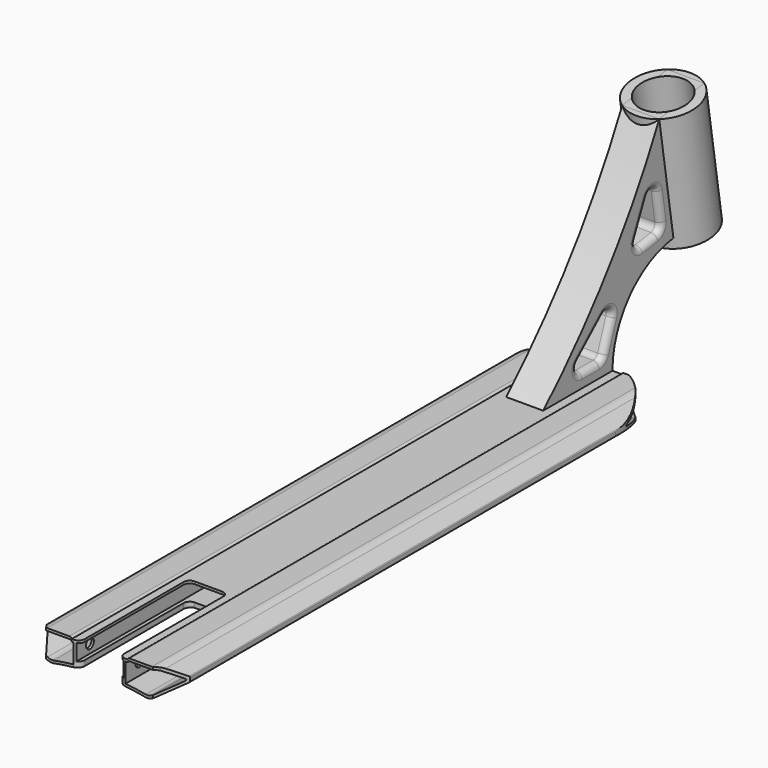
from build123d import *

# Parameters (mm, degrees)
F1_DEPTH       = 250
F2_W           = 38
F2_H           = 13
F3_DEPTH       = 250
F4_R           = 9
F5_R           = 1
F6_T1_DEPTH    = 509.3674969976
F8_DEPTH       = 500.001
F10_DEPTH      = 526
F10_DEPTH_BACK = 24.001
F12_DEPTH      = 527
F12_DEPTH_BACK = 24.0010001
F13_F1_R       = 4.9999
F13_F2_R       = 5
F13_F3_R       = 5
F13_F4_R       = 4.9999
F13_F5_R       = 5
F13_F6_R       = 5
F15_DEPTH      = 15
F16_R          = 27.5
F17_DEPTH      = 100
F19_D          = 40
F21_D          = 8
F21_DEPTH      = 50
F21_TIP        = 2.4034424761
F23_DEPTH      = 72.5010001
F24_R          = 5


# Not quite as in the source:
# - a fillet or chamfer that OpenCascade refuses, or shapes differently, is made with other operations: its cross-section is extruded or revolved along the edge and cut away or added
# - a fillet or chamfer is up to 0.001 mm smaller than in the source, because OpenCascade refuses the exact size
# - an extrude ends at something that could not be found from the text; its depth is read off the source's solid


with BuildPart() as f1:
    # F0 (on Front) → F1 (new body, symmetric)
    with BuildSketch(Plane.XZ):
        with BuildLine():
            Line((22.5, 22.7), (0, 22.7))
            Line((0, 22.7), (-22.5, 22.7))
            Line((-22.5, 22.7), (-22.5, 24))
            Line((-22.5, 24), (-45.5824640741, 24))
            Line((-45.5824640741, 24), (-57.5, 14))
            Line((-57.5, 14), (-57.5, 10))
            Line((-57.5, 10), (-40.1794919243, 0))
            ThreePointArc((-40.1794919243, 0), (0, 4.0775448584), (40.1794919243, 0))
            Line((40.1794919243, 0), (57.5, 10))
            Line((57.5, 10), (57.5, 14))
            Line((57.5, 14), (45.5824640741, 24))
            Line((45.5824640741, 24), (22.5, 24))
            Line((22.5, 24), (22.5, 22.7))
        make_face()
    extrude(amount=F1_DEPTH, both=True)

    # F2 (on Front) → F3 (cut, symmetric)
    with BuildSketch(Plane.XZ):
        with Locations((0, 14.2)):
            Rectangle(F2_W, F2_H)
    extrude(amount=F3_DEPTH, both=True, mode=Mode.SUBTRACT)

    # F4
    f4_edges = [f1.edges().sort_by_distance(p)[0] for p in [
        (40.179492, 0, 0),
        (-40.179492, 0, 0),
        (-45.582464, 0, 24),
        (45.582464, 0, 24),
    ]]
    fillet(f4_edges, radius=F4_R)

    # F5
    f5_edges = [f1.edges().sort_by_distance(p)[0] for p in [
        (57.5, 0, 14),
        (57.5, 0, 10),
        (-57.5, 0, 14),
        (-57.5, 0, 10),
    ]]
    fillet(f5_edges, radius=F5_R)

    # F6: fillet of radius 2 on 2 edges, made by hand

    # F6_s2 → F6_t1 (cut)
    with BuildSketch(Plane.XZ.offset(-254.6837484988)):
        with BuildLine():
            ThreePointArc((-22.5, 22.7), (-23.2333239744, 23.6431676725), (-24.3734993995, 24))
            Line((-24.3734993995, 24), (-22.5, 24))
            Line((-22.5, 24), (-22.5, 22.7))
        make_face()
        with BuildLine():
            ThreePointArc((24.3734993995, 24), (23.2333239744, 23.6431676725), (22.5, 22.7))
            Line((22.5, 22.7), (22.5, 24))
            Line((22.5, 24), (24.3734993995, 24))
        make_face()
    extrude(amount=F6_T1_DEPTH, mode=Mode.SUBTRACT)

    # F7 (on face) → F8 (cut, through all)
    with BuildSketch(Plane.XZ.offset(250)):
        with BuildLine():
            Line((-24.3734993995, 22), (-42.3067319657, 22))
            ThreePointArc((-42.3067319657, 22), (-44.7008729689, 21.5778483455), (-46.8062452335, 20.3623111018))
            Line((-46.8062452335, 20.3623111018), (-55.7563117574, 12.8523135826))
            ThreePointArc((-55.7563117574, 12.8523135826), (-56.1097188459, 11.9991133967), (-55.6135241478, 11.2202437356))
            Line((-55.6135241478, 11.2202437356), (-42.1022690923, 3.4195169923))
            ThreePointArc((-42.1022690923, 3.4195169923), (-39.7790673433, 2.5813219392), (-37.3093701274, 2.6021299876))
            ThreePointArc((-37.3093701274, 2.6021299876), (-29.1789785809, 3.9589777355), (-21, 4.9829952574))
            Line((-21, 4.9829952574), (-21, 20.7))
            Line((-21, 20.7), (-22.5, 20.7))
            ThreePointArc((-22.5, 20.7), (-23.2333239744, 21.6431676725), (-24.3734993995, 22))
        make_face()
        with BuildLine():
            Line((21, 20.7), (21, 4.9829952574))
            ThreePointArc((21, 4.9829952574), (29.1789785809, 3.9589777355), (37.3093701274, 2.6021299876))
            ThreePointArc((37.3093701274, 2.6021299876), (39.7790673433, 2.5813219392), (42.1022690923, 3.4195169923))
            Line((42.1022690923, 3.4195169923), (55.6135241478, 11.2202437356))
            ThreePointArc((55.6135241478, 11.2202437356), (56.1097188459, 11.9991133967), (55.7563117574, 12.8523135826))
            Line((55.7563117574, 12.8523135826), (46.8062452335, 20.3623111018))
            ThreePointArc((46.8062452335, 20.3623111018), (44.7008729689, 21.5778483455), (42.3067319657, 22))
            Line((42.3067319657, 22), (24.3734993995, 22))
            ThreePointArc((24.3734993995, 22), (23.2333239744, 21.6431676725), (22.5, 20.7))
            Line((22.5, 20.7), (21, 20.7))
        make_face()
    extrude(amount=-F8_DEPTH, mode=Mode.SUBTRACT)

    # F9 (on Top) → F10 (cut, two sides)
    with BuildSketch(Plane.XY) as f10_sk:
        with BuildLine():
            ThreePointArc((-57.5, 200), (0, 257.5), (57.5, 200))
            Line((57.5, 200), (57.5, 280))
            Line((57.5, 280), (-57.5, 280))
            Line((-57.5, 280), (-57.5, 200))
        make_face()
    extrude(amount=-F10_DEPTH, mode=Mode.SUBTRACT)
    extrude(f10_sk.sketch, amount=F10_DEPTH_BACK, mode=Mode.SUBTRACT)

    # F11 (on Top) → F12 (cut, two sides)
    with BuildSketch(Plane.XY) as f12_sk:
        Polygon((-43.2975540478, -250), (-68, -216), (-68, -346), (68, -346), (68, -216), (43.2975540478, -250), (16, -250), (16, -140), (-16, -140), (-16, -250), align=None)
    extrude(amount=-F12_DEPTH, mode=Mode.SUBTRACT)
    extrude(f12_sk.sketch, amount=F12_DEPTH_BACK, mode=Mode.SUBTRACT)

    # F13: fillet of radius 5 on 8 edges, made by hand

    # F13_f1 (radius 5 in the source; OpenCascade refuses exactly that, so slightly less here)
    f13_f1_edges = [f1.edges().sort_by_distance(p)[0] for p in [
        (16, -250, 5.5682587842),
    ]]
    fillet(f13_f1_edges, radius=F13_F1_R)

    # F13_f2
    f13_f2_edges = [f1.edges().sort_by_distance(p)[0] for p in [
        (16, -140, 5.5682587842),
    ]]
    fillet(f13_f2_edges, radius=F13_F2_R)

    # F13_f3
    f13_f3_edges = [f1.edges().sort_by_distance(p)[0] for p in [
        (16, -140, 21.7),
    ]]
    fillet(f13_f3_edges, radius=F13_F3_R)

    # F13_f4 (radius 5 in the source; OpenCascade refuses exactly that, so slightly less here)
    f13_f4_edges = [f1.edges().sort_by_distance(p)[0] for p in [
        (-16, -250, 21.7),
    ]]
    fillet(f13_f4_edges, radius=F13_F4_R)

    # F13_f5
    f13_f5_edges = [f1.edges().sort_by_distance(p)[0] for p in [
        (-16, -140, 5.5682587842),
    ]]
    fillet(f13_f5_edges, radius=F13_F5_R)

    # F13_f6
    f13_f6_edges = [f1.edges().sort_by_distance(p)[0] for p in [
        (-16, -140, 21.7),
    ]]
    fillet(f13_f6_edges, radius=F13_F6_R)

    # F14 (on Right) → F15 (join, symmetric)
    with BuildSketch(Plane.YZ):
        with BuildLine():
            ThreePointArc((297.3819995028, 182.7), (245.9666940414, 97.362277853), (180, 22.7))
            Line((180, 22.7), (250, 22.7))
            ThreePointArc((250, 22.7), (267.6550746197, 69.1758946867), (311.7145367693, 92.2079211245))
            Line((311.7145367693, 92.2079211245), (313.0254460068, 83.9311659405))
            Line((313.0254460068, 83.9311659405), (358.4591096742, 91.1271513323))
            Line((358.4591096742, 91.1271513323), (342.8156631702, 189.8959853919))
            Line((342.8156631702, 189.8959853919), (297.3819995028, 182.7))
        make_face()
    extrude(amount=F15_DEPTH, both=True)

    # F16 (on face) → F17 (join, through all)
    with BuildSketch(Plane(origin=(0, -20.9512469128, 132.2809669298), x_dir=(1, 0, 0), z_dir=(0, -0.156434465, 0.9876883406))):
        with Locations((0, 345.3013103746)):
            Circle(F16_R)
    extrude(amount=-F17_DEPTH)

    # F19 (through all)
    with Locations(Plane(origin=(0, -20.9512469128, 132.2809669298), x_dir=(1, 0, 0), z_dir=(0, -0.156434465, 0.9876883406))):
        with Locations((0, 345.3013103746)):
            Hole(F19_D / 2)

    # F21 (one way)
    with BuildSketch(Plane.YZ.offset(21)):
        with Locations((-236, 14.9829952574)):
            Circle(F21_D / 2)
    extrude(amount=-F21_DEPTH, mode=Mode.SUBTRACT)
    with Locations(Plane.YZ.offset(21)):
        with Locations((-236, 14.9829952574)):
            with Locations((0, 0, -(F21_DEPTH + F21_TIP / 2))):  # 118° drill point
                Cone(0, F21_D / 2, F21_TIP, mode=Mode.SUBTRACT)

    # F22 (on face) → F23 (cut, through all)
    with BuildSketch(Plane.YZ.offset(15)):
        Polygon((292.844313904, 147.1129445351), (270.3409635007, 97.4199105839), (299.9716137186, 102.1129445351), align=None)
        Polygon((256.378660542, 79), (206, 34), (240, 34), align=None)
    extrude(amount=-F23_DEPTH, mode=Mode.SUBTRACT)

    # F24
    f24_edges = [f1.edges().sort_by_distance(p)[0] for p in [
        (15, 248.18933, 56.5),
        (0, 256.378661, 79),
        (-15, 248.18933, 56.5),
        (0, 240, 34),
        (15, 296.407964, 124.612945),
        (0, 292.844314, 147.112945),
        (-15, 296.407964, 124.612945),
        (0, 299.971614, 102.112945),
        (15, 281.592639, 122.266428),
        (0, 270.340964, 97.419911),
        (-15, 281.592639, 122.266428),
        (15, 231.18933, 56.5),
        (0, 206, 34),
        (-15, 231.18933, 56.5),
        (15, 223, 34),
        (-15, 223, 34),
        (15, 285.156289, 99.766428),
        (-15, 285.156289, 99.766428),
    ]]
    fillet(f24_edges, radius=F24_R)


solid = f1.part
